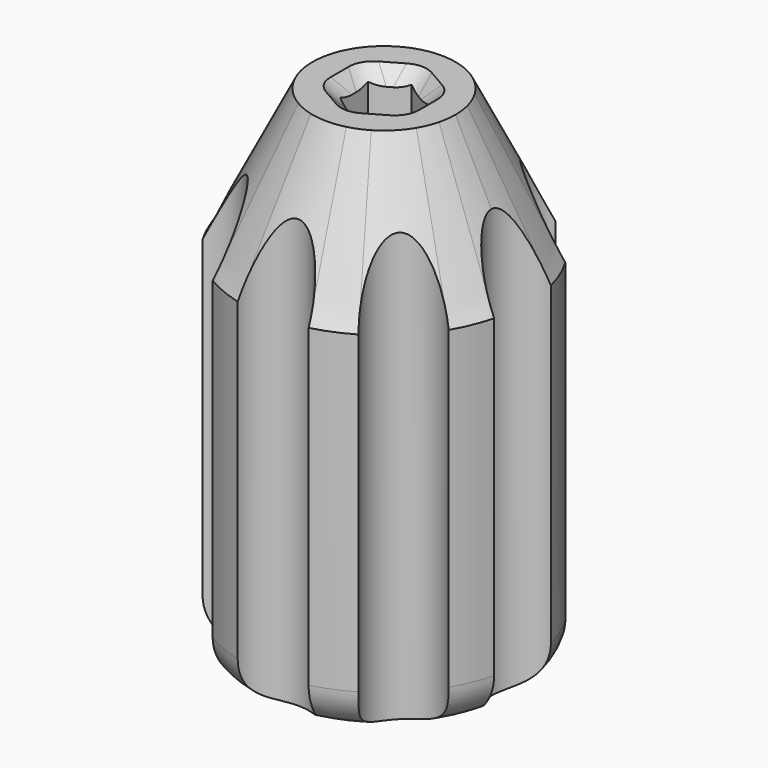
from build123d import *

# Parameters (mm, degrees)
F1_DEPTH = 35
F2_DEPTH = 25
F3_R     = 3
F4_SIZE2 = 5
F4_SIZE  = 10
F5_SIZE  = 1
F6_R     = 2.5
F7_DEPTH = 40


# Not quite as in the source:
# - a feature names something its author has since deleted; it is built from what else it names


with BuildPart() as f1:
    # F0 (on Top) → F1 (new body)
    with BuildSketch(Plane.XY):
        with BuildLine():
            ThreePointArc((9.6875, -2.4803918541), (7.5, 0), (9.6875, 2.4803918541))
            ThreePointArc((9.6875, 2.4803918541), (9.2387953251, 3.8268343237), (8.6039988428, 5.0961950427))
            ThreePointArc((8.6039988428, 5.0961950427), (5.3033008589, 5.3033008589), (5.0961950427, 8.6039988428))
            ThreePointArc((5.0961950427, 8.6039988428), (3.8268343237, 9.2387953251), (2.4803918541, 9.6875))
            ThreePointArc((2.4803918541, 9.6875), (0, 7.5), (-2.4803918541, 9.6875))
            ThreePointArc((-2.4803918541, 9.6875), (-3.8268343237, 9.2387953251), (-5.0961950427, 8.6039988428))
            ThreePointArc((-5.0961950427, 8.6039988428), (-4.7059904428, 7.8812585539), (-4.5710678119, 7.0710678119))
            ThreePointArc((-4.5710678119, 7.0710678119), (-5.971596934, 4.8258141984), (-8.6039988428, 5.0961950427))
            ThreePointArc((-8.6039988428, 5.0961950427), (-9.2387953251, 3.8268343237), (-9.6875, 2.4803918541))
            ThreePointArc((-9.6875, 2.4803918541), (-8.125, 1.6535945694), (-7.5, 0))
            ThreePointArc((-7.5, 0), (-8.125, -1.6535945694), (-9.6875, -2.4803918541))
            ThreePointArc((-9.6875, -2.4803918541), (-9.2387953251, -3.8268343237), (-8.6039988428, -5.0961950427))
            ThreePointArc((-8.6039988428, -5.0961950427), (-5.971596934, -4.8258141984), (-4.5710678119, -7.0710678119))
            ThreePointArc((-4.5710678119, -7.0710678119), (-4.7059904428, -7.8812585539), (-5.0961950427, -8.6039988428))
            ThreePointArc((-5.0961950427, -8.6039988428), (-3.8268343237, -9.2387953251), (-2.4803918541, -9.6875))
            ThreePointArc((-2.4803918541, -9.6875), (0, -7.5), (2.4803918541, -9.6875))
            ThreePointArc((2.4803918541, -9.6875), (3.8268343237, -9.2387953251), (5.0961950427, -8.6039988428))
            ThreePointArc((5.0961950427, -8.6039988428), (5.3033008589, -5.3033008589), (8.6039988428, -5.0961950427))
            ThreePointArc((8.6039988428, -5.0961950427), (9.2387953251, -3.8268343237), (9.6875, -2.4803918541))
        make_face()
        Polygon((0, 2.4248711306), (2.1, 1.2124355653), (2.1, -1.2124355653), (0, -2.4248711306), (-2.1, -1.2124355653), (-2.1, 1.2124355653), align=None, mode=Mode.SUBTRACT)
        with BuildLine():
            ThreePointArc((-2.4803918541, 9.6875), (0, 7.5), (2.4803918541, 9.6875))
            ThreePointArc((2.4803918541, 9.6875), (0, 10), (-2.4803918541, 9.6875))
        make_face()
        with BuildLine():
            ThreePointArc((-8.6039988428, -5.0961950427), (-7.0710678119, -7.0710678119), (-5.0961950427, -8.6039988428))
            ThreePointArc((-5.0961950427, -8.6039988428), (-4.7059904428, -7.8812585539), (-4.5710678119, -7.0710678119))
            ThreePointArc((-4.5710678119, -7.0710678119), (-5.971596934, -4.8258141984), (-8.6039988428, -5.0961950427))
        make_face()
        with BuildLine():
            ThreePointArc((-7.5, 0), (-8.125, 1.6535945694), (-9.6875, 2.4803918541))
            ThreePointArc((-9.6875, 2.4803918541), (-10, 0), (-9.6875, -2.4803918541))
            ThreePointArc((-9.6875, -2.4803918541), (-8.125, -1.6535945694), (-7.5, 0))
        make_face()
        with BuildLine():
            ThreePointArc((-2.4803918541, -9.6875), (0, -10), (2.4803918541, -9.6875))
            ThreePointArc((2.4803918541, -9.6875), (0, -7.5), (-2.4803918541, -9.6875))
        make_face()
        with BuildLine():
            ThreePointArc((5.0961950427, -8.6039988428), (7.0710678119, -7.0710678119), (8.6039988428, -5.0961950427))
            ThreePointArc((8.6039988428, -5.0961950427), (5.3033008589, -5.3033008589), (5.0961950427, -8.6039988428))
        make_face()
        with BuildLine():
            ThreePointArc((9.6875, -2.4803918541), (9.9215674165, -1.25), (10, 0))
            ThreePointArc((10, 0), (9.9215674165, 1.25), (9.6875, 2.4803918541))
            ThreePointArc((9.6875, 2.4803918541), (7.5, 0), (9.6875, -2.4803918541))
        make_face()
        with BuildLine():
            ThreePointArc((5.0961950427, 8.6039988428), (5.3033008589, 5.3033008589), (8.6039988428, 5.0961950427))
            ThreePointArc((8.6039988428, 5.0961950427), (7.0710678119, 7.0710678119), (5.0961950427, 8.6039988428))
        make_face()
        with BuildLine():
            ThreePointArc((-4.5710678119, 7.0710678119), (-4.7059904428, 7.8812585539), (-5.0961950427, 8.6039988428))
            ThreePointArc((-5.0961950427, 8.6039988428), (-7.0710678119, 7.0710678119), (-8.6039988428, 5.0961950427))
            ThreePointArc((-8.6039988428, 5.0961950427), (-5.971596934, 4.8258141984), (-4.5710678119, 7.0710678119))
        make_face()
    extrude(amount=F1_DEPTH)

    # F0 (on Top) → F2 (join)
    with BuildSketch(Plane.XY):
        Polygon((2.1, -1.2124355653), (2.1, 1.2124355653), (0, 2.4248711306), (-2.1, 1.2124355653), (-2.1, -1.2124355653), (0, -2.4248711306), align=None)
    extrude(amount=F2_DEPTH)

    # F3
    f3_edges = [f1.edges().sort_by_distance(p)[0] for p in [
        (5.096195, -8.603999, 0),
    ]]
    fillet(f3_edges, radius=F3_R)

    # F4
    f4_edges = [f1.edges().sort_by_distance(p)[0] for p in [
        (5.096195, -8.603999, 35),
    ]]
    f4_side = f1.faces().sort_by_distance((5.096195, -8.603999, 19))[0]
    chamfer(f4_edges, length=F4_SIZE, length2=F4_SIZE2, reference=f4_side)

    # F5
    f5_edges = [f1.edges().sort_by_distance(p)[0] for p in [
        (1.05, -1.818653, 35),
        (2.1, 0, 35),
        (1.05, 1.818653, 35),
        (-1.05, 1.818653, 35),
        (-2.1, 0, 35),
        (-1.05, -1.818653, 35),
    ]]
    chamfer(f5_edges, length=F5_SIZE)

    # F6
    f6_edges = [f1.edges().sort_by_distance(p)[0] for p in [
        (0, 3.002221, 34.5),
        (2.6, 1.501111, 34.5),
        (2.6, -1.501111, 34.5),
        (0, -3.002221, 34.5),
        (-2.6, -1.501111, 34.5),
        (-2.6, 1.501111, 34.5),
    ]]
    fillet(f6_edges, radius=F6_R)

    # F0 (on Top) → F7 (cut)
    with BuildSketch(Plane.XY):
        with BuildLine():
            ThreePointArc((-8.6039988428, -5.0961950427), (-7.0710678119, -7.0710678119), (-5.0961950427, -8.6039988428))
            ThreePointArc((-5.0961950427, -8.6039988428), (-4.7059904428, -7.8812585539), (-4.5710678119, -7.0710678119))
            ThreePointArc((-4.5710678119, -7.0710678119), (-5.971596934, -4.8258141984), (-8.6039988428, -5.0961950427))
        make_face()
        with BuildLine():
            ThreePointArc((-2.4803918541, 9.6875), (0, 7.5), (2.4803918541, 9.6875))
            ThreePointArc((2.4803918541, 9.6875), (0, 10), (-2.4803918541, 9.6875))
        make_face()
        with BuildLine():
            ThreePointArc((-4.5710678119, 7.0710678119), (-4.7059904428, 7.8812585539), (-5.0961950427, 8.6039988428))
            ThreePointArc((-5.0961950427, 8.6039988428), (-7.0710678119, 7.0710678119), (-8.6039988428, 5.0961950427))
            ThreePointArc((-8.6039988428, 5.0961950427), (-5.971596934, 4.8258141984), (-4.5710678119, 7.0710678119))
        make_face()
        with BuildLine():
            ThreePointArc((-7.5, 0), (-8.125, 1.6535945694), (-9.6875, 2.4803918541))
            ThreePointArc((-9.6875, 2.4803918541), (-10, 0), (-9.6875, -2.4803918541))
            ThreePointArc((-9.6875, -2.4803918541), (-8.125, -1.6535945694), (-7.5, 0))
        make_face()
        with BuildLine():
            ThreePointArc((-2.4803918541, -9.6875), (0, -10), (2.4803918541, -9.6875))
            ThreePointArc((2.4803918541, -9.6875), (0, -7.5), (-2.4803918541, -9.6875))
        make_face()
        with BuildLine():
            ThreePointArc((5.0961950427, -8.6039988428), (7.0710678119, -7.0710678119), (8.6039988428, -5.0961950427))
            ThreePointArc((8.6039988428, -5.0961950427), (5.3033008589, -5.3033008589), (5.0961950427, -8.6039988428))
        make_face()
        with BuildLine():
            ThreePointArc((9.6875, -2.4803918541), (9.9215674165, -1.25), (10, 0))
            ThreePointArc((10, 0), (9.9215674165, 1.25), (9.6875, 2.4803918541))
            ThreePointArc((9.6875, 2.4803918541), (7.5, 0), (9.6875, -2.4803918541))
        make_face()
        with BuildLine():
            ThreePointArc((5.0961950427, 8.6039988428), (5.3033008589, 5.3033008589), (8.6039988428, 5.0961950427))
            ThreePointArc((8.6039988428, 5.0961950427), (7.0710678119, 7.0710678119), (5.0961950427, 8.6039988428))
        make_face()
    extrude(amount=F7_DEPTH, mode=Mode.SUBTRACT)


solid = f1.part
